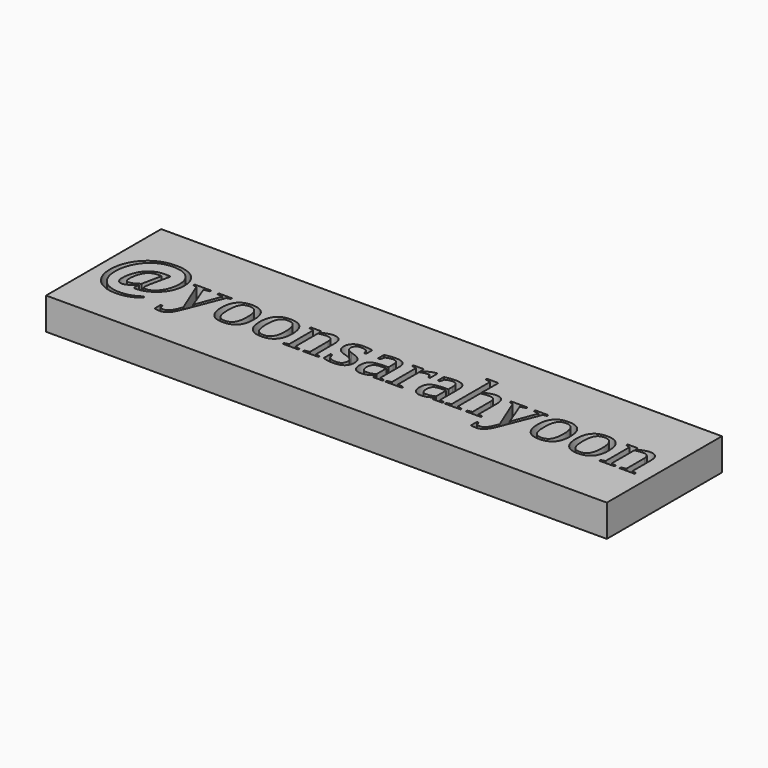
from build123d import *

# Parameters (mm, degrees)
F0_W         = 35.0933708251
F0_H         = 9.0042063966
F1_DEPTH     = 2
F2_TEXT_SIZE = 4.8175653016
F3_DEPTH     = 2


# Not quite as in the source:
# - Text() gives the source's letters only with a copy of the font that has no kerning and outlines rounded to 1/6400 em; it was checked with that copy


with BuildPart() as f1:
    # F0 (on Top) → F1 (new body)
    with BuildSketch(Plane.XY):
        Rectangle(F0_W, F0_H)
    extrude(amount=F1_DEPTH)

    # F2 (on face) → F3 (cut)
    with BuildSketch(Plane.XY.offset(2)):
        with Locations((-17.0934732596, -1.2672713365)):
            Text('@yoonsarahyoon', F2_TEXT_SIZE, font='Tinos', text_align=(TextAlign.LEFT, TextAlign.BOTTOM))
    extrude(amount=-F3_DEPTH, mode=Mode.SUBTRACT)


solid = f1.part
